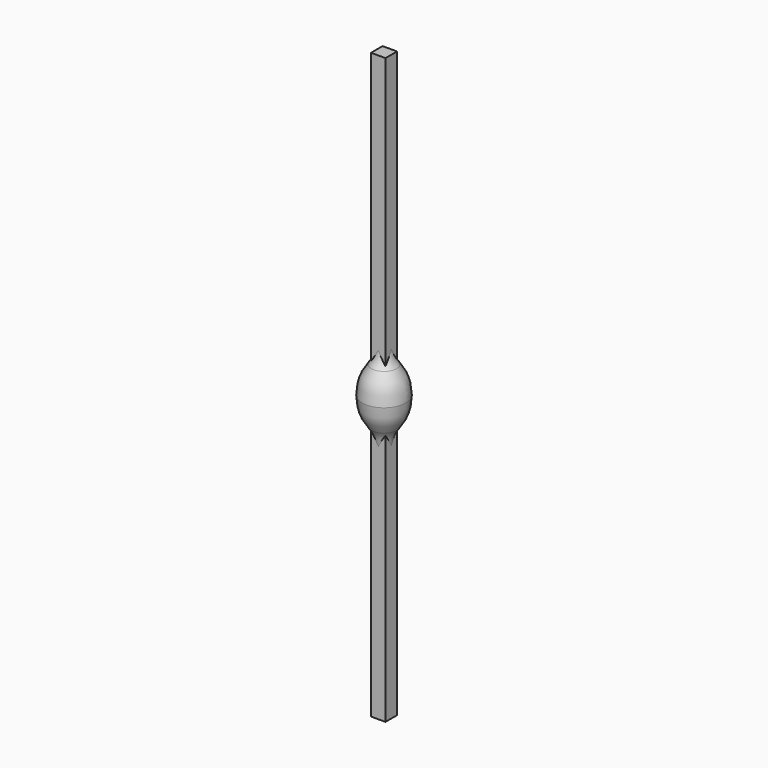
from build123d import *

# Parameters (mm, degrees)
F3_DEPTH      = 210
F3_DEPTH_BACK = 25
F5_DEPTH      = 194
F5_DEPTH_BACK = 25


with BuildPart() as f1:
    # F0 (on Front) → F1 (revolve)
    with BuildSketch(Plane.XZ):
        with BuildLine():
            Line((6, 40), (0, 40))
            Line((0, 40), (0, -40))
            Line((0, -40), (6, -40))
            Line((6, -40), (6, -35))
            ThreePointArc((6, -35), (7.121945325, -28.3955279025), (10.3619051686, -22.5320414644))
            ThreePointArc((10.3619051686, -22.5320414644), (16.1478700246, -11.9337677658), (17.9879737223, 0))
            ThreePointArc((17.9879737223, 0), (16.1478700246, 11.9337677658), (10.3619051686, 22.5320414644))
            ThreePointArc((10.3619051686, 22.5320414644), (7.121945325, 28.3955279025), (6, 35))
            Line((6, 35), (6, 40))
        make_face()
    revolve(axis=Axis((0, 0, 0), (0, 0, -1)))

    # F2 (on face) → F3 (join, two sides)
    with BuildSketch(Plane.XY.offset(40)) as f3_sk:
        with BuildLine():
            Line((6, 0), (6, 6))
            Line((6, 6), (0, 6))
            ThreePointArc((0, 6), (4.2426406871, 4.2426406871), (6, 0))
        make_face()
        with BuildLine():
            ThreePointArc((-6, 0), (-4.2426406871, 4.2426406871), (0, 6))
            Line((0, 6), (-6, 6))
            Line((-6, 6), (-6, 0))
        make_face()
        with BuildLine():
            ThreePointArc((0, -6), (-4.2426406871, -4.2426406871), (-6, 0))
            Line((-6, 0), (-6, -6))
            Line((-6, -6), (0, -6))
        make_face()
        with BuildLine():
            Line((6, -6), (6, 0))
            ThreePointArc((6, 0), (4.2426406871, -4.2426406871), (0, -6))
            Line((0, -6), (6, -6))
        make_face()
        with BuildLine():
            ThreePointArc((6, 0), (4.2426406871, 4.2426406871), (0, 6))
            ThreePointArc((0, 6), (-4.2426406871, 4.2426406871), (-6, 0))
            ThreePointArc((-6, 0), (-4.2426406871, -4.2426406871), (0, -6))
            ThreePointArc((0, -6), (4.2426406871, -4.2426406871), (6, 0))
        make_face()
    extrude(amount=F3_DEPTH)
    extrude(f3_sk.sketch, amount=-F3_DEPTH_BACK)

    # F4 (on face) → F5 (join, two sides)
    with BuildSketch(Plane(origin=(0, 0, -40), x_dir=(1, 0, 0), z_dir=(0, 0, -1))) as f5_sk:
        with BuildLine():
            Line((6, 0), (6, 6))
            Line((6, 6), (0, 6))
            ThreePointArc((0, 6), (4.2426406871, 4.2426406871), (6, 0))
        make_face()
        with BuildLine():
            ThreePointArc((-6, 0), (-4.2426406871, 4.2426406871), (0, 6))
            Line((0, 6), (-6, 6))
            Line((-6, 6), (-6, 0))
        make_face()
        with BuildLine():
            ThreePointArc((6, 0), (4.2426406871, 4.2426406871), (0, 6))
            ThreePointArc((0, 6), (-4.2426406871, 4.2426406871), (-6, 0))
            ThreePointArc((-6, 0), (-4.2426406871, -4.2426406871), (0, -6))
            ThreePointArc((0, -6), (4.2426406871, -4.2426406871), (6, 0))
        make_face()
        with BuildLine():
            Line((6, -6), (6, 0))
            ThreePointArc((6, 0), (4.2426406871, -4.2426406871), (0, -6))
            Line((0, -6), (6, -6))
        make_face()
        with BuildLine():
            ThreePointArc((0, -6), (-4.2426406871, -4.2426406871), (-6, 0))
            Line((-6, 0), (-6, -6))
            Line((-6, -6), (0, -6))
        make_face()
    extrude(amount=F5_DEPTH)
    extrude(f5_sk.sketch, amount=-F5_DEPTH_BACK)


solid = f1.part
